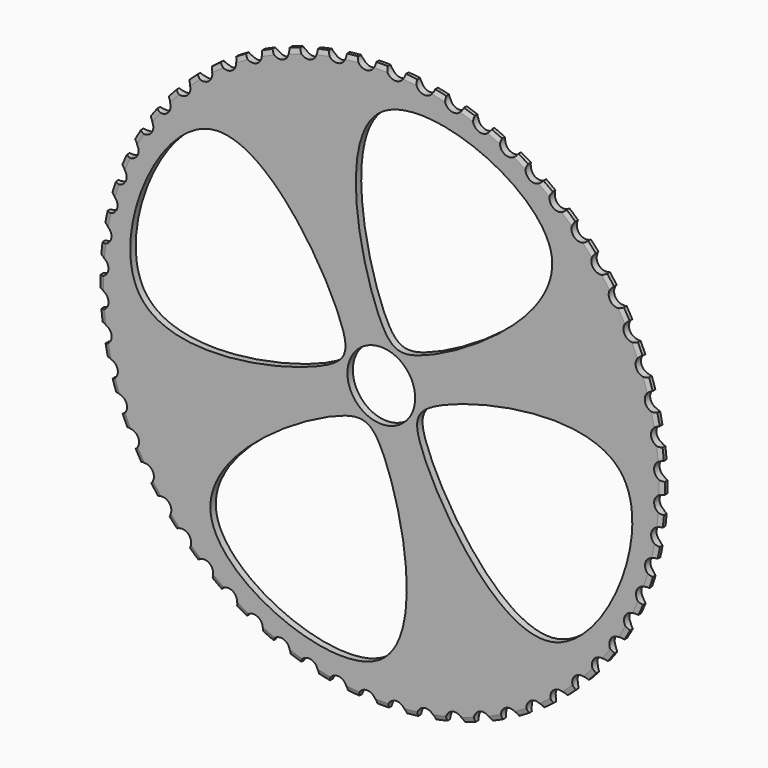
from build123d import *

# Parameters (mm, degrees)
F0_R     = 125
F1_DEPTH = 3
F2_SIZE2 = 2
F2_SIZE  = 0.75
F5_DEPTH = 3.001
F4_R     = 4
F4_R_2   = 15
F6_DEPTH = 3.0010001


# Not quite as in the source:
# - two fillets or chamfers of one size are made in one step


with BuildPart() as f1:
    # F0 (on Front) → F1 (new body)
    with BuildSketch(Plane.XZ):
        Circle(F0_R)
    extrude(amount=F1_DEPTH)

    # F2
    f2_edges = [f1.edges().sort_by_distance(p)[0] for p in [
        (-125, 0, 0),
        (-125, -3, 0),
    ]]
    f2_side = f1.faces().sort_by_distance((-125, -1.5, 0))[0]
    chamfer(f2_edges, length=F2_SIZE, length2=F2_SIZE2, reference=f2_side)

    # F4 (on face) → F5 (cut, through all)
    with BuildSketch(Plane.XZ.offset(3)):
        with BuildLine():
            ThreePointArc((-111.2094421684, 52.5495953608), (-109.6980974197, 55.6356668199), (-108.1011346438, 58.6783153195))
            ThreePointArc((-108.1011346438, 58.6783153195), (-108.7666163141, 59.4776138408), (-109.6156692621, 60.0783243127))
            ThreePointArc((-109.6156692621, 60.0783243127), (-111.4818063209, 56.5403118088), (-113.23378601, 52.9444020256))
            ThreePointArc((-113.23378601, 52.9444020256), (-112.24749791, 52.6142811938), (-111.2094421684, 52.5495953608))
        make_face()
        with BuildLine():
            ThreePointArc((-113.23378601, 52.9444020256), (-111.4818063209, 56.5403118088), (-109.6156692621, 60.0783243127))
            ThreePointArc((-109.6156692621, 60.0783243127), (-115.0492241231, 58.3496017867), (-113.23378601, 52.9444020256))
        make_face()
    extrude(amount=-F5_DEPTH, mode=Mode.SUBTRACT)

    # F4 (on face) → F6 (cut, through all)
    with BuildSketch(Plane.XZ.offset(3)):
        with Locations((-111.4818063209, 56.5403118088)):
            Circle(F4_R)
        with Locations((-116.7811692274, 44.5775561678)):
            Circle(F4_R)
        with Locations((-120.8010532058, 32.1263994929)):
            Circle(F4_R)
        with Locations((-123.497415566, 19.3232592624)):
            Circle(F4_R)
        with Locations((-124.8407143978, 6.3084093597)):
            Circle(F4_R)
        with Locations((-124.816232238, -6.7755567961)):
            Circle(F4_R)
        with Locations((-123.4242373184, -19.7852885337)):
            Circle(F4_R)
        with Locations((-120.6799806266, -32.5782485099)):
            Circle(F4_R)
        with Locations((-116.6135288131, -45.0142743779)):
            Circle(F4_R)
        with Locations((-111.2694347749, -56.957114436)):
            Circle(F4_R)
        with Locations((-104.7062495248, -68.2759204292)):
            Circle(F4_R)
        with Locations((-96.9958806936, -78.8466811506)):
            Circle(F4_R)
        with Locations((-88.2228046959, -88.5535811336)):
            Circle(F4_R)
        with Locations((-78.4831411881, -97.2902695507)):
            Circle(F4_R)
        with Locations((-67.8835999618, -104.9610254153)):
            Circle(F4_R)
        with Locations((-56.5403118088, -111.4818063209)):
            Circle(F4_R)
        with Locations((-44.5775561678, -116.7811692274)):
            Circle(F4_R)
        with Locations((-32.1263994929, -120.8010532058)):
            Circle(F4_R)
        with Locations((-19.3232592624, -123.497415566)):
            Circle(F4_R)
        with Locations((-6.3084093597, -124.8407143978)):
            Circle(F4_R)
        with Locations((6.7755567961, -124.816232238)):
            Circle(F4_R)
        with Locations((19.7852885337, -123.4242373184)):
            Circle(F4_R)
        with Locations((32.5782485099, -120.6799806266)):
            Circle(F4_R)
        with Locations((45.0142743779, -116.6135288131)):
            Circle(F4_R)
        with Locations((56.957114436, -111.2694347749)):
            Circle(F4_R)
        with Locations((68.2759204292, -104.7062495248)):
            Circle(F4_R)
        with Locations((78.8466811506, -96.9958806936)):
            Circle(F4_R)
        with Locations((88.5535811336, -88.2228046959)):
            Circle(F4_R)
        with Locations((97.2902695507, -78.4831411881)):
            Circle(F4_R)
        with Locations((104.9610254153, -67.8835999618)):
            Circle(F4_R)
        with Locations((111.4818063209, -56.5403118088)):
            Circle(F4_R)
        with Locations((116.7811692274, -44.5775561678)):
            Circle(F4_R)
        with Locations((120.8010532058, -32.1263994929)):
            Circle(F4_R)
        with Locations((123.497415566, -19.3232592624)):
            Circle(F4_R)
        with Locations((124.8407143978, -6.3084093597)):
            Circle(F4_R)
        with Locations((124.816232238, 6.7755567961)):
            Circle(F4_R)
        with Locations((123.4242373184, 19.7852885337)):
            Circle(F4_R)
        with Locations((120.6799806266, 32.5782485099)):
            Circle(F4_R)
        with Locations((116.6135288131, 45.0142743779)):
            Circle(F4_R)
        with Locations((111.2694347749, 56.957114436)):
            Circle(F4_R)
        with Locations((104.7062495248, 68.2759204292)):
            Circle(F4_R)
        with Locations((96.9958806936, 78.8466811506)):
            Circle(F4_R)
        with Locations((88.2228046959, 88.5535811336)):
            Circle(F4_R)
        with Locations((78.4831411881, 97.2902695507)):
            Circle(F4_R)
        with Locations((67.8835999618, 104.9610254153)):
            Circle(F4_R)
        with Locations((56.5403118088, 111.4818063209)):
            Circle(F4_R)
        with Locations((44.5775561678, 116.7811692274)):
            Circle(F4_R)
        with Locations((32.1263994929, 120.8010532058)):
            Circle(F4_R)
        with Locations((19.3232592624, 123.497415566)):
            Circle(F4_R)
        with Locations((6.3084093597, 124.8407143978)):
            Circle(F4_R)
        with Locations((-6.7755567961, 124.816232238)):
            Circle(F4_R)
        with Locations((-19.7852885337, 123.4242373184)):
            Circle(F4_R)
        with Locations((-32.5782485099, 120.6799806266)):
            Circle(F4_R)
        with Locations((-45.0142743779, 116.6135288131)):
            Circle(F4_R)
        with Locations((-56.957114436, 111.2694347749)):
            Circle(F4_R)
        with Locations((-68.2759204292, 104.7062495248)):
            Circle(F4_R)
        with Locations((-78.8466811506, 96.9958806936)):
            Circle(F4_R)
        with Locations((-88.5535811336, 88.2228046959)):
            Circle(F4_R)
        with Locations((-97.2902695507, 78.4831411881)):
            Circle(F4_R)
        with Locations((-104.9610254153, 67.8835999618)):
            Circle(F4_R)
        Circle(F4_R_2)
        with BuildLine():
            add(Edge.make_bspline(
                [(-106.6350535542, 0), (-120.7426065525, 20.0632613723), (-78.3262241543, 122.465467025), (-10.9071572344, 16.1074401319), (-19.1022049887, -3.6771553009), (-92.4870405073, -20.1208022178), (-106.6350535542, 0)],
                knots=[0, 0, 0, 0, 0.2868974632, 0.5746177399, 0.7122797233, 1, 1, 1, 1], degree=3))
        make_face()
        with BuildLine():
            add(Edge.make_bspline(
                [(0, 106.6350535542), (20.0632613723, 120.7426065525), (122.465467025, 78.3262241543), (16.1074401319, 10.9071572344), (-3.6771553009, 19.1022049887), (-20.1208022178, 92.4870405073), (0, 106.6350535542)],
                knots=[0, 0, 0, 0, 0.2868974632, 0.5746177399, 0.7122797233, 1, 1, 1, 1], degree=3))
        make_face()
        with BuildLine():
            add(Edge.make_bspline(
                [(106.6350535542, 0), (120.7426065525, -20.0632613723), (78.3262241543, -122.465467025), (10.9071572344, -16.1074401319), (19.1022049887, 3.6771553009), (92.4870405073, 20.1208022178), (106.6350535542, 0)],
                knots=[0, 0, 0, 0, 0.2868974632, 0.5746177399, 0.7122797233, 1, 1, 1, 1], degree=3))
        make_face()
        with BuildLine():
            add(Edge.make_bspline(
                [(0, -106.6350535542), (-20.0632613723, -120.7426065525), (-122.465467025, -78.3262241543), (-16.1074401319, -10.9071572344), (3.6771553009, -19.1022049887), (20.1208022178, -92.4870405073), (0, -106.6350535542)],
                knots=[0, 0, 0, 0, 0.2868974632, 0.5746177399, 0.7122797233, 1, 1, 1, 1], degree=3))
        make_face()
    extrude(amount=-F6_DEPTH, mode=Mode.SUBTRACT)


solid = f1.part
